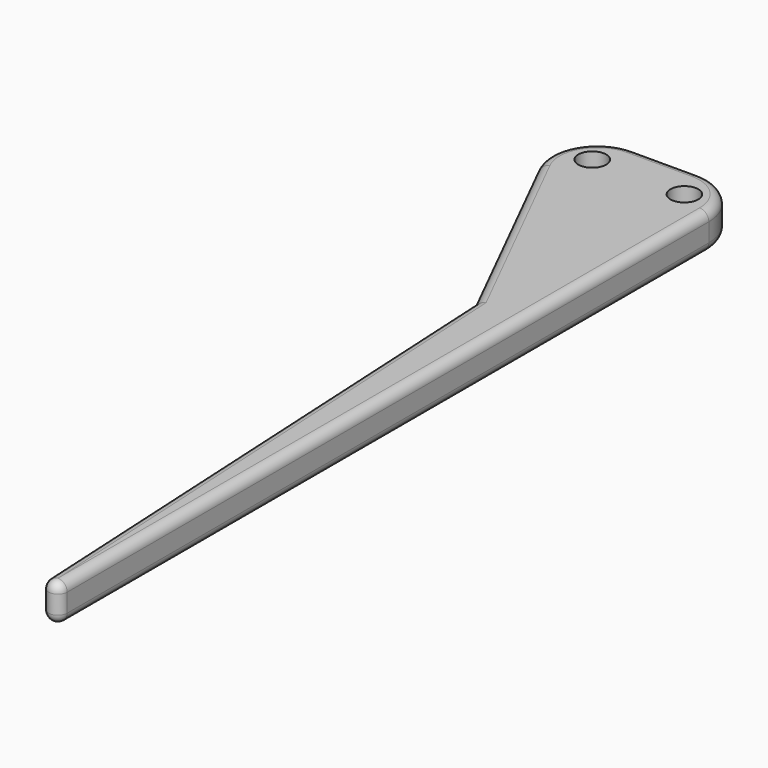
from build123d import *

# Parameters (mm, degrees)
F1_DEPTH = 4
F2_R     = 5.08
F3_R     = 5.08
F4_R     = 1
F5_R     = 1
F6_R     = 1.5
F7_DEPTH = 25.4
F8_R     = 1


# Not quite as in the source:
# - a feature names something its author has since deleted; it is built from what else it names


with BuildPart() as f1:
    # F0 (on Top) → F1 (new body)
    with BuildSketch(Plane.XY):
        Polygon((0, -130), (0, 0), (-20.2767271549, 0), (-5.2268992042, -30.1366958052), align=None)
    extrude(amount=F1_DEPTH)

    # F2
    f2_edges = [f1.edges().sort_by_distance(p)[0] for p in [
        (0, 0, 2),
    ]]
    fillet(f2_edges, radius=F2_R)

    # F3
    f3_edges = [f1.edges().sort_by_distance(p)[0] for p in [
        (-20.276727, 0, 2),
    ]]
    fillet(f3_edges, radius=F3_R)

    # F4
    f4_edges = [f1.edges().sort_by_distance(p)[0] for p in [
        (0, -130, 2),
    ]]
    fillet(f4_edges, radius=F4_R)

    # F5
    f5_edges = [f1.edges().sort_by_distance(p)[0] for p in [
        (-10.916669, -18.743153, 4),
        (-3.612766, -60.975757, 4),
    ]]
    fillet(f5_edges, radius=F5_R)

    # F6 (on face) → F7 (cut)
    with BuildSketch(Plane.XY.offset(4)):
        with Locations((-13.589, -3.840335412)):
            Circle(F6_R)
        with Locations((-3.5482854582, -3.9438293315)):
            Circle(F6_R)
    extrude(amount=-F7_DEPTH, mode=Mode.SUBTRACT)

    # F8
    f8_edges = [f1.edges().sort_by_distance(p)[0] for p in [
        (-8.570816, 0, 0),
        (-10.916669, -18.743153, 0),
    ]]
    fillet(f8_edges, radius=F8_R)


solid = f1.part
